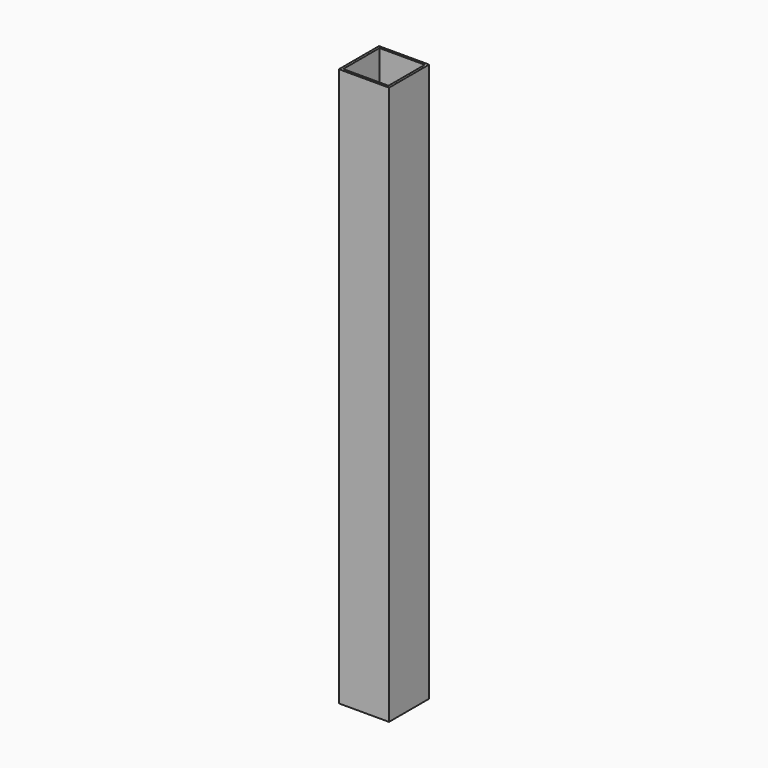
from build123d import *

# Parameters (mm, degrees)
F0_W     = 63.5
F0_H     = 63.5
F0_W_2   = 57.5
F0_H_2   = 57.5
F1_DEPTH = 705


# Not quite as in the source:
# - a pattern or mirror of a feature is missing from the dataset's text; its kind, count and spacing are read off the source's solid


with BuildPart() as f1:
    # F0 (on Top) → F1 (new body)
    with BuildSketch(Plane.XY):
        with Locations((5.787525326, -9.6492074422)):
            Rectangle(F0_W, F0_H)
        with Locations((5.787525326, -9.6492074422)):
            Rectangle(F0_W_2, F0_H_2, mode=Mode.SUBTRACT)
    extrude(amount=F1_DEPTH)

    # F1_copies: F1 across plane


with BuildPart() as f1_1:
    add(f1.part)
    add(f1.part.mirror(Plane.XY.offset(354)))


solid = f1_1.part
